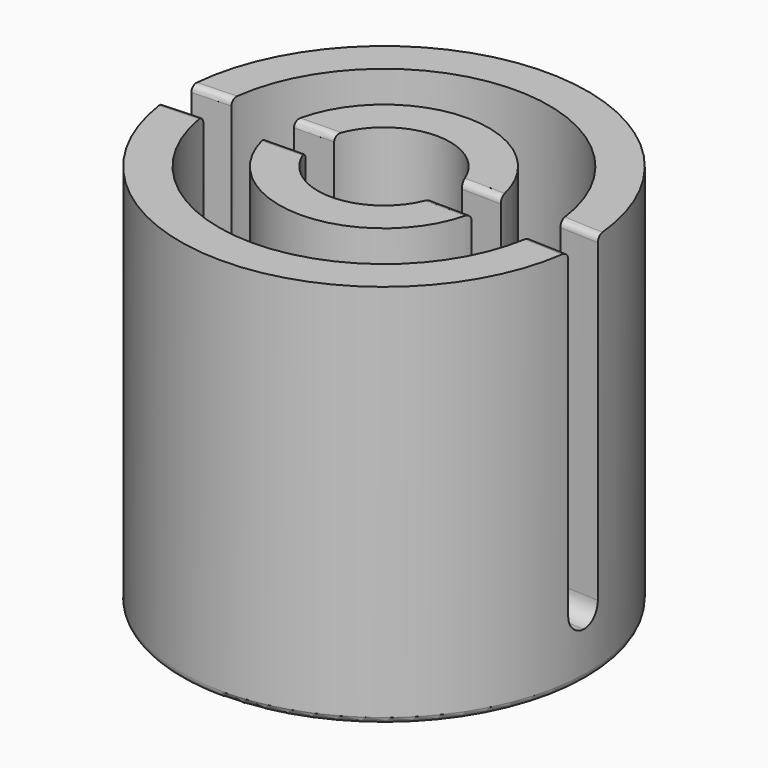
from build123d import *

# Parameters (mm, degrees)
F0_R      = 15.85
F0_R_2    = 5.15
F1_DEPTH  = 30
F2_R      = 12.85
F2_R_2    = 8.15
F3_DEPTH  = 40
F4_R      = 12.65
F4_R_2    = 8.9
F5_DEPTH  = 40
F10_R     = 0.5
F11_R     = 15.35
F12_DEPTH = 3


# Not quite as in the source:
# - a feature names something its author has since deleted; it is built from what else it names


with BuildPart() as f1:
    # F0 (on Top) → F1 (new body)
    with BuildSketch(Plane.XY):
        Circle(F0_R)
        Circle(F0_R_2, mode=Mode.SUBTRACT)
    extrude(amount=F1_DEPTH)

    # F2 (on face) → F3 (cut)
    with BuildSketch(Plane.XY.offset(30)):
        Circle(F2_R)
        Circle(F2_R_2, mode=Mode.SUBTRACT)
    extrude(amount=-F3_DEPTH, mode=Mode.SUBTRACT)

    # F4 (on face) → F5 (cut)
    with BuildSketch(Plane(origin=(0, 0, 0), x_dir=(1, 0, 0), z_dir=(0, 0, -1))):
        Circle(F4_R)
        Circle(F4_R_2, mode=Mode.SUBTRACT)
    extrude(amount=-F5_DEPTH, mode=Mode.SUBTRACT)

    # F7 (on Right) → F9 (revolve, cut)
    with BuildSketch(Plane.YZ):
        with BuildLine():
            Line((1.4, 5), (1.4, 30))
            Line((1.4, 30), (0, 30))
            Line((0, 30), (-1.4, 30))
            Line((-1.4, 30), (-1.4, 5))
            ThreePointArc((-1.4, 5), (-0.9899494937, 4.0100505063), (0, 3.6))
            ThreePointArc((0, 3.6), (0.9899494937, 4.0100505063), (1.4, 5))
        make_face()
    revolve(axis=Axis((0, -340, 29.7196172178), (0, 0, 1)), mode=Mode.SUBTRACT)

    # F10
    f10_edges = [f1.edges().sort_by_distance(p)[0] for p in [
        (-14.307042, 1.100086, 30),
        (14.307042, 1.100086, 30),
        (6.50553, 1.338011, 30),
        (-6.50553, 1.338011, 30),
        (14.248226, -1.699914, 30),
        (-14.248226, -1.699914, 30),
        (-6.478795, -1.461989, 30),
        (6.478795, -1.461989, 30),
        (-15.85, 0, 0),
    ]]
    fillet(f10_edges, radius=F10_R)

    # F11 (on face) → F12 (join)
    with BuildSketch(Plane(origin=(0, 0, 0), x_dir=(1, 0, 0), z_dir=(0, 0, -1))):
        Circle(F11_R)
    extrude(amount=-F12_DEPTH)


solid = f1.part
